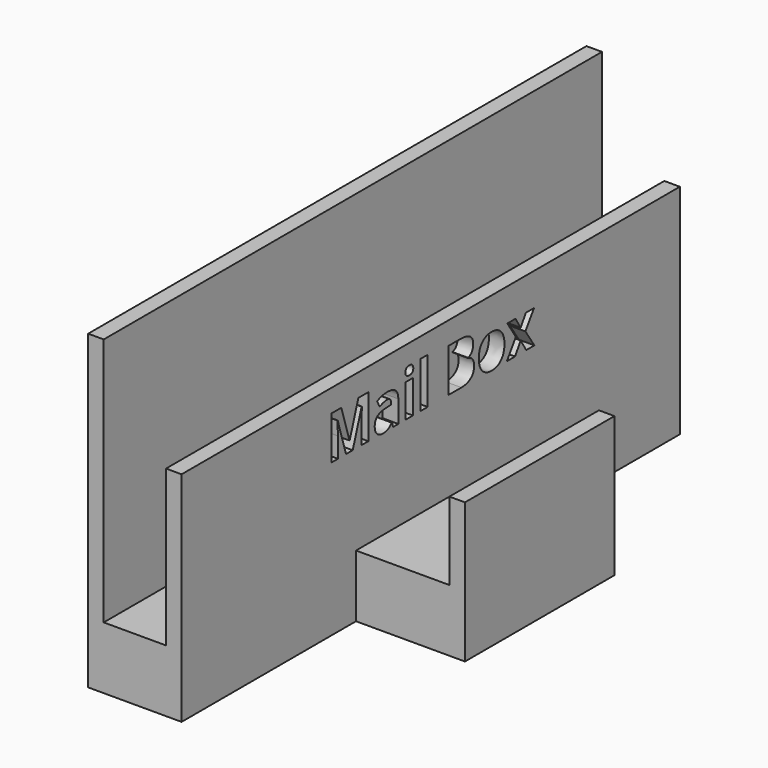
from build123d import *

# Parameters (mm, degrees)
F2_DEPTH     = 200
F3_W         = 40.0817116683
F3_H         = 60.1724977605
F4_DEPTH     = 70
F8_TEXT_SIZE = 19.4444444444
F9_DEPTH     = 5


# Not quite as in the source:
# - Text() gives the source's letters only with a copy of the font that has no kerning and outlines rounded to 1/6400 em; it was checked with that copy


with BuildPart() as f2:
    # F1 (on Front) → F2 (new body)
    with BuildSketch(Plane.XZ):
        Polygon((-26.8333567679, 100), (-31.8333567679, 100), (-31.8333567679, 0), (33.1666432321, 0), (33.1666432321, 45), (28.1666432321, 45), (28.1666432321, 20), (-1.8333567679, 20), (-1.8333567679, 70), (-6.8333567679, 70), (-6.8333567679, 20), (-26.8333567679, 20), align=None)
    extrude(amount=F2_DEPTH)


with BuildPart() as f4:
    # F3 (on Front) → F4 (new body)
    with BuildSketch(Plane.XZ):
        with Locations((18.2074990663, 26.1507222895)):
            Rectangle(F3_W, F3_H)
    extrude(amount=F4_DEPTH)


with BuildPart() as f6_1:
    # F6: instance of F4
    add(f4.part.mirror(Plane(origin=(-3.9116700209, -100, 25.2108433735), x_dir=(1, 0, 0), z_dir=(0, -1, 0))))


with BuildPart() as f2_1:
    add(f2.part)

    # F7: cut F6_1, F4
    add(f6_1.part, mode=Mode.SUBTRACT)
    add(f4.part, mode=Mode.SUBTRACT)

    # F8 (on face) → F9 (cut)
    with BuildSketch(Plane.YZ.offset(-1.8333567679)):
        with BuildLine():
            add(Edge.make_bspline(
                [(-77.2243923611, 56.572630422), (-77.7378472222, 55.7887762553), (-77.7378472222, 54.2028387553)],
                knots=[0, 0, 0, 1, 1, 1], degree=2))
            add(Edge.make_bspline(
                [(-77.7378472222, 54.2028387553), (-77.7378472222, 52.6260158386), (-77.2198350694, 51.8193752136)],
                knots=[0, 0, 0, 1, 1, 1], degree=2))
            add(Edge.make_bspline(
                [(-77.2198350694, 51.8193752136), (-76.7018229167, 51.0127345886), (-75.53515625, 51.0127345886)],
                knots=[0, 0, 0, 1, 1, 1], degree=2))
            add(Edge.make_bspline(
                [(-75.53515625, 51.0127345886), (-74.3745659722, 51.0127345886), (-73.8671875, 51.814817922)],
                knots=[0, 0, 0, 1, 1, 1], degree=2))
            add(Edge.make_bspline(
                [(-73.8671875, 51.814817922), (-73.3598090278, 52.6169012553), (-73.3598090278, 54.2028387553)],
                knots=[0, 0, 0, 1, 1, 1], degree=2))
            add(Edge.make_bspline(
                [(-73.3598090278, 54.2028387553), (-73.3598090278, 55.779661672), (-73.8717447917, 56.5680731303)],
                knots=[0, 0, 0, 1, 1, 1], degree=2))
            add(Edge.make_bspline(
                [(-73.8717447917, 56.5680731303), (-74.3836805556, 57.3564845886), (-75.5533854167, 57.3564845886)],
                knots=[0, 0, 0, 1, 1, 1], degree=2))
            add(Edge.make_bspline(
                [(-75.5533854167, 57.3564845886), (-76.7109375, 57.3564845886), (-77.2243923611, 56.572630422)],
                knots=[0, 0, 0, 1, 1, 1], degree=2))
        make_face()
        with BuildLine():
            Line((-88.11328125, 54.9259290331), (-89.9361979167, 54.9259290331))
            Line((-89.9361979167, 54.9259290331), (-89.9361979167, 51.3074394498))
            Line((-89.9361979167, 51.3074394498), (-88.0190972222, 51.3074394498))
            add(Edge.make_bspline(
                [(-88.0190972222, 51.3074394498), (-86.8038194444, 51.3074394498), (-86.2250434028, 51.7722831998)],
                knots=[0, 0, 0, 1, 1, 1], degree=2))
            add(Edge.make_bspline(
                [(-86.2250434028, 51.7722831998), (-85.6462673611, 52.2371269498), (-85.6462673611, 53.1971963942)],
                knots=[0, 0, 0, 1, 1, 1], degree=2))
            add(Edge.make_bspline(
                [(-85.6462673611, 53.1971963942), (-85.6462673611, 54.9259290331), (-88.11328125, 54.9259290331)],
                knots=[0, 0, 0, 1, 1, 1], degree=2))
        make_face()
        with BuildLine():
            Line((-89.9361979167, 60.346067922), (-89.9361979167, 57.2592623664))
            Line((-89.9361979167, 57.2592623664), (-88.2287326389, 57.2592623664))
            add(Edge.make_bspline(
                [(-88.2287326389, 57.2592623664), (-87.0316840278, 57.2592623664), (-86.4954427083, 57.6299220886)],
                knots=[0, 0, 0, 1, 1, 1], degree=2))
            add(Edge.make_bspline(
                [(-86.4954427083, 57.6299220886), (-85.9592013889, 58.0005818109), (-85.9592013889, 58.8543144498)],
                knots=[0, 0, 0, 1, 1, 1], degree=2))
            add(Edge.make_bspline(
                [(-85.9592013889, 58.8543144498), (-85.9592013889, 59.6533595886), (-86.5425347222, 59.9997137553)],
                knots=[0, 0, 0, 1, 1, 1], degree=2))
            add(Edge.make_bspline(
                [(-86.5425347222, 59.9997137553), (-87.1258680556, 60.346067922), (-88.3897569444, 60.346067922)],
                knots=[0, 0, 0, 1, 1, 1], degree=2))
            Line((-88.3897569444, 60.346067922), (-89.9361979167, 60.346067922))
        make_face()
        with BuildLine():
            Line((-115.8854166667, 52.9207206998), (-115.8854166667, 53.7957206998))
            Line((-115.8854166667, 53.7957206998), (-117.0065104167, 53.756224172))
            add(Edge.make_bspline(
                [(-117.0065104167, 53.756224172), (-118.2703993056, 53.7197658386), (-118.8871527778, 53.3020141025)],
                knots=[0, 0, 0, 1, 1, 1], degree=2))
            add(Edge.make_bspline(
                [(-118.8871527778, 53.3020141025), (-119.50390625, 52.8842623664), (-119.50390625, 52.0305297275)],
                knots=[0, 0, 0, 1, 1, 1], degree=2))
            add(Edge.make_bspline(
                [(-119.50390625, 52.0305297275), (-119.50390625, 50.803099172), (-118.1002604167, 50.803099172)],
                knots=[0, 0, 0, 1, 1, 1], degree=2))
            add(Edge.make_bspline(
                [(-118.1002604167, 50.803099172), (-117.0915798611, 50.803099172), (-116.4884982639, 51.3833943109)],
                knots=[0, 0, 0, 1, 1, 1], degree=2))
            add(Edge.make_bspline(
                [(-116.4884982639, 51.3833943109), (-115.8854166667, 51.9636894498), (-115.8854166667, 52.9207206998)],
                knots=[0, 0, 0, 1, 1, 1], degree=2))
        make_face()
        with Locations((-141.625, 48.8768838942)):
            Text('Mail Box', F8_TEXT_SIZE, font='Open Sans', font_style=FontStyle.BOLD, text_align=(TextAlign.LEFT, TextAlign.BOTTOM))
    extrude(amount=-F9_DEPTH, mode=Mode.SUBTRACT)


solid = f2_1.part
